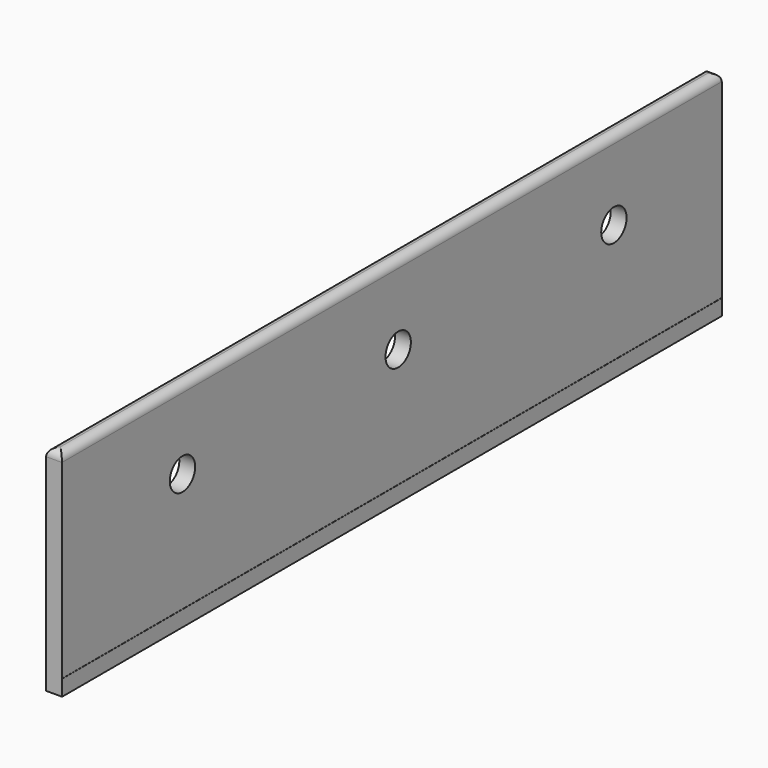
from build123d import *

# Parameters (mm, degrees)
F0_W      = 104
F0_H      = 104
F1_DEPTH  = 2
F2_W      = 2
F2_H      = 104
F3_DEPTH  = 25
F4_W      = 2
F4_H      = 104
F5_DEPTH  = 25
F6_R      = 0.99999
F7_R      = 0.99999
F9_D      = 4
F11_D     = 4
F13_D     = 4
F15_DEPTH = 500
F16_DEPTH = 505


# Not quite as in the source:
# - a fillet or chamfer is up to 0.001 mm smaller than in the source, because OpenCascade refuses the exact size


with BuildPart() as f1:
    # F0 (on Top) → F1 (new body)
    with BuildSketch(Plane.XY):
        Rectangle(F0_W, F0_H)
    extrude(amount=F1_DEPTH)

    # F2 (on face) → F3 (join)
    with BuildSketch(Plane.XY.offset(2)):
        with Locations((-51, 0)):
            Rectangle(F2_W, F2_H)
    extrude(amount=F3_DEPTH)

    # F4 (on face) → F5 (join)
    with BuildSketch(Plane.XY.offset(2)):
        with Locations((51, 0)):
            Rectangle(F4_W, F4_H)
    extrude(amount=F5_DEPTH)

    # F6 (radius 1 in the source; OpenCascade refuses exactly that, so slightly less here)
    f6_edges = [f1.edges().sort_by_distance(p)[0] for p in [
        (52, 0, 27),
        (51, 52, 27),
        (50, 0, 27),
        (51, -52, 27),
    ]]
    fillet(f6_edges, radius=F6_R)

    # F7 (radius 1 in the source; OpenCascade refuses exactly that, so slightly less here)
    f7_edges = [f1.edges().sort_by_distance(p)[0] for p in [
        (-51, 52, 27),
        (-52, 0, 27),
        (-51, -52, 27),
        (-50, 0, 27),
    ]]
    fillet(f7_edges, radius=F7_R)

    # F9 (through all)
    with Locations(Plane.YZ.offset(52)):
        with Locations((-33, 17)):
            Hole(F9_D / 2)

    # F11 (through all)
    with Locations(Plane.YZ.offset(52)):
        with Locations((1, 17)):
            Hole(F11_D / 2)

    # F13 (through all)
    with Locations(Plane.YZ.offset(52)):
        with Locations((35, 17)):
            Hole(F13_D / 2)

    # F14 (on Front) → F15 (cut)
    with BuildSketch(Plane.XZ):
        Polygon((74.380248785, 39.0327088535), (-49.979981035, 2.7150458191), (-49.979981035, 0), (-49.979981035, -1.495702425), (74.380248785, -1.495702425), align=None)
    extrude(amount=F15_DEPTH, mode=Mode.SUBTRACT)

    # F14 (on Front) → F16 (cut)
    with BuildSketch(Plane.XZ):
        Polygon((74.380248785, 39.0327088535), (-49.979981035, 2.7150458191), (-49.979981035, 0), (-49.979981035, -1.495702425), (74.380248785, -1.495702425), align=None)
    extrude(amount=-F16_DEPTH, mode=Mode.SUBTRACT)


solid = f1.part
